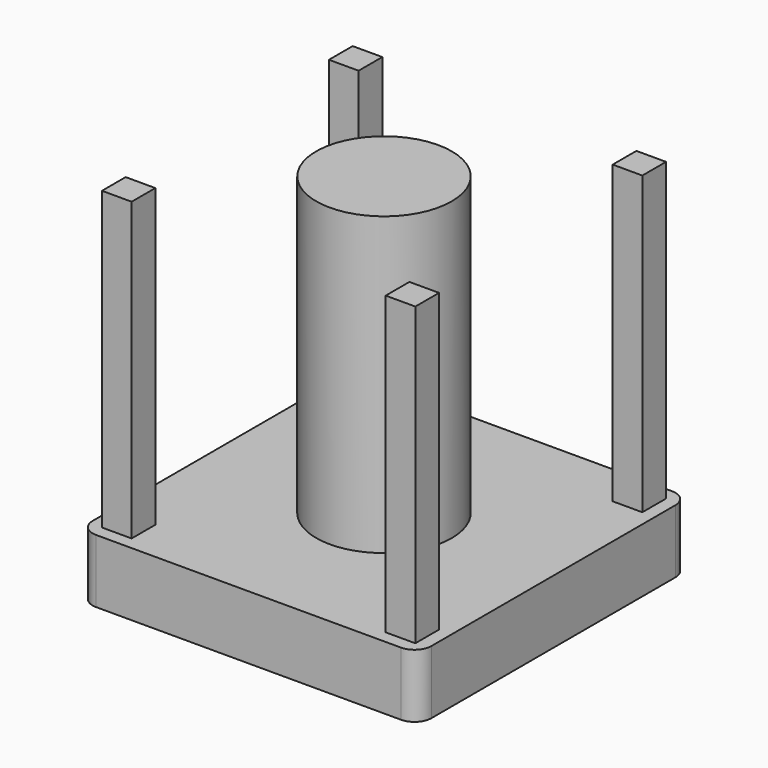
from build123d import *

# Parameters (mm, degrees)
F0_W     = 101.6
F0_H     = 101.6
F1_DEPTH = 19.05
F3_DEPTH = 88.9
F4_R     = 20.32
F5_DEPTH = 88.9
F6_R     = 5.08
F7_R     = 5.08
F8_R     = 5.08
F9_R     = 5.08


# Not quite as in the source:
# - the program builds the solid bodies; features that only make, move or delete a surface that nothing else refers to are left out


with BuildPart() as f1:
    # F0 (on Top) → F1 (new body)
    with BuildSketch(Plane.XY):
        Rectangle(F0_W, F0_H)
    extrude(amount=-F1_DEPTH)

    # F6
    f6_edges = [f1.edges().sort_by_distance(p)[0] for p in [
        (-50.8, 50.8, -9.525),
    ]]
    fillet(f6_edges, radius=F6_R)

    # F7
    f7_edges = [f1.edges().sort_by_distance(p)[0] for p in [
        (50.8, 50.8, -9.525),
    ]]
    fillet(f7_edges, radius=F7_R)

    # F8
    f8_edges = [f1.edges().sort_by_distance(p)[0] for p in [
        (50.8, -50.8, -9.525),
    ]]
    fillet(f8_edges, radius=F8_R)

    # F9
    f9_edges = [f1.edges().sort_by_distance(p)[0] for p in [
        (-50.8, -50.8, -9.525),
    ]]
    fillet(f9_edges, radius=F9_R)


with BuildPart() as f3:
    # F2 (on face) → F3 (new body)
    with BuildSketch(Plane.XY):
        Polygon((42.291, -38.1), (38.1, -38.1), (38.1, -42.291), (38.1, -42.799), (38.1, -46.99), (46.99, -46.99), (46.99, -38.1), (42.799, -38.1), align=None)
    extrude(amount=F3_DEPTH)


with BuildPart() as f3b:
    # F2 (on face) → F3, piece 2 (new body)
    with BuildSketch(Plane.XY):
        Polygon((-38.1, -42.799), (-38.1, -42.291), (-38.1, -38.1), (-42.291, -38.1), (-42.799, -38.1), (-44.1724389358, -38.1), (-44.6804389358, -38.1), (-46.99, -38.1), (-46.99, -46.99), (-38.1, -46.99), align=None)
    extrude(amount=F3_DEPTH)


with BuildPart() as f3c:
    # F2 (on face) → F3, piece 3 (new body)
    with BuildSketch(Plane.XY):
        Polygon((-38.1, 38.1), (-38.1, 42.291), (-38.1, 42.799), (-38.1, 46.99), (-46.99, 46.99), (-46.99, 38.1), (-44.6804389358, 38.1), (-44.1724389358, 38.1), (-42.799, 38.1), (-42.291, 38.1), align=None)
    extrude(amount=F3_DEPTH)


with BuildPart() as f3d:
    # F2 (on face) → F3, piece 4 (new body)
    with BuildSketch(Plane.XY):
        Polygon((38.1, 38.1), (42.291, 38.1), (42.799, 38.1), (46.99, 38.1), (46.99, 46.99), (38.1, 46.99), (38.1, 42.799), (38.1, 42.291), align=None)
    extrude(amount=F3_DEPTH)


with BuildPart() as f5:
    # F4 (on face) → F5 (new body)
    with BuildSketch(Plane.XY):
        Circle(F4_R)
    extrude(amount=F5_DEPTH)


solid = Compound([f1.part, f3.part, f3b.part, f3c.part, f3d.part, f5.part])
